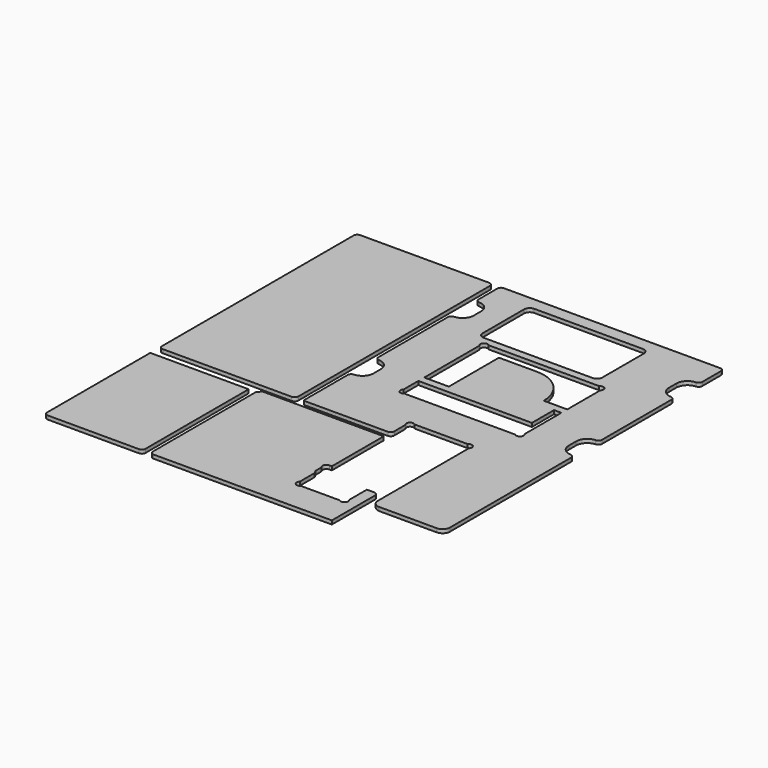
from build123d import *

# Parameters (mm, degrees)
F1_DEPTH = 1


# Not quite as in the source:
# - ends of sketch curves that miss each other by under 0.0002 mm in the source are joined


with BuildPart() as f1:
    # F0 (on Top) → F1 (new body)
    with BuildSketch(Plane.XY):
        with BuildLine():
            Line((-49.84369, 52.000023), (-49.84369, -4.632071))
            Line((-49.84369, -4.632071), (-49.84369, -12.999847))
            ThreePointArc((-49.84369, -12.999847), (-49.5508014675, -13.7069564675), (-48.843692, -13.999845))
            Line((-48.843692, -13.999845), (-13.843762, -13.999845))
            ThreePointArc((-13.843762, -13.9998449989), (-13.136642867, -13.706966133), (-12.8437640011, -12.999847))
            Line((-12.843764, -12.999847), (-12.843764, -4.632071))
            Line((-12.843764, -4.632071), (-12.843764, 52.000023))
            ThreePointArc((-12.8437640013, 52.000023), (-13.1366419884, 52.7071430116), (-13.843762, 53.0000209987))
            Line((-13.843762, 53.000021), (-48.843692, 53.000021))
            ThreePointArc((-48.843692, 53.0000209998), (-49.5508026391, 52.7071336391), (-49.8436899998, 52.000023))
        make_face()
    extrude(amount=F1_DEPTH)


with BuildPart() as f1b:
    # F0 (on Top) → F1, piece 2 (new body)
    with BuildSketch(Plane.XY):
        with BuildLine():
            Line((-48.843692, -53.000021), (-24.125936, -53.000021))
            ThreePointArc((-24.125936, -53.000021), (-23.4188315117, -52.7071274883), (-23.125938, -52.000023))
            Line((-23.125938, -52.000023), (-23.125938, -16.999839))
            Line((-23.125938, -16.999839), (-49.84369, -16.999839))
            Line((-49.84369, -16.999839), (-49.84369, -52.000023))
            ThreePointArc((-49.843689999, -52.000023), (-49.5507844797, -52.7071154797), (-48.843692, -53.000020999))
        make_face()
    extrude(amount=F1_DEPTH)


with BuildPart() as f1c:
    # F0 (on Top) → F1, piece 3 (new body)
    with BuildSketch(Plane.XY):
        with BuildLine():
            ThreePointArc((11.3220496611, -35.3140013389), (11.1054475003, -34.2240151152), (12.0297310005, -33.6070171613))
            Line((12.0297310005, -33.6070171613), (12.722098, -33.607018))
            Line((12.722098, -33.607018), (12.722098, -15.999841))
            Line((12.722098, -15.999841), (-20.125944, -15.999841))
            Line((-20.125944, -15.999841), (-21.125942, -16.999839))
            Line((-21.125942, -16.999839), (-21.125942, -52.000023))
            ThreePointArc((-21.125942, -52.000023), (-20.8330265213, -52.7071055213), (-20.125944, -53.000020997))
            Line((-20.125944, -53.000020997), (28.242006, -53.000021))
            Line((28.242006, -53.000021), (28.242006, -52.000023))
            Line((28.242006, -52.000023), (28.242006, -38.339903))
            ThreePointArc((28.242006, -38.339903), (27.9606950958, -37.6445668865), (27.2750267787, -37.3404499772))
            Line((27.2750267787, -37.3404499772), (25.221946, -37.341683))
            Line((25.221946, -37.341683), (25.221946, -43.335575))
            ThreePointArc((25.221946, -43.335575), (25.2219457726, -44.7498467726), (23.8076742274, -44.7498467726))
            Line((23.8076742274, -44.7498467726), (13.236194, -44.749847))
            ThreePointArc((13.236194, -44.749847), (11.8219222274, -44.7498467726), (11.8219222274, -43.3355752274))
            Line((11.8219222274, -43.3355752274), (11.821922, -38.348793))
            Line((11.821922, -38.348793), (11.8126693234, -38.3302876467))
            Line((11.8126693234, -38.3302876467), (11.3316786766, -37.3683063533))
            Line((11.3316786766, -37.3683063533), (11.32205, -37.349049))
            Line((11.32205, -37.349049), (11.3220496611, -35.3140013389))
        make_face()
    extrude(amount=F1_DEPTH)


with BuildPart() as f1d:
    # F0 (on Top) → F1, piece 4 (new body)
    with BuildSketch(Plane.XY):
        with BuildLine():
            Line((-9.84377, -13.814933), (12.077446, -13.814933))
            ThreePointArc((12.077446, -13.814933), (12.7580726434, -13.5084192102), (13.0368039831, -12.815951))
            Line((13.0368039831, -12.815951), (13.036804, -9.064371))
            ThreePointArc((13.036804, -9.064371), (13.0368846628, -7.6501796628), (14.4510763316, -7.6503526685))
            Line((14.4510763316, -7.6503526685), (28.82773, -7.650353))
            ThreePointArc((28.82773, -7.650353), (30.2419053372, -7.6501956628), (30.2420023393, -9.0643713393))
            Line((30.2420023393, -9.0643713393), (30.242002, -39.915465))
            ThreePointArc((30.242002, -39.915465), (30.8277878518, -41.3296751482), (32.241998, -41.915461))
            Line((32.241998, -41.915461), (47.843694, -41.915461))
            ThreePointArc((47.843694, -41.915461), (49.2579050268, -41.3296760268), (49.84369, -39.915465))
            Line((49.84369, -39.915465), (49.84369, 1.188847))
            ThreePointArc((49.84369, 1.188847), (49.5650323815, 1.8814639379), (48.8843320024, 2.1880830581))
            ThreePointArc((48.8843320024, 2.1880830581), (46.8422776076, 3.1078090407), (46.0062580004, 5.185537))
            Line((46.0062580004, 5.185537), (46.006258, 7.685405))
            ThreePointArc((46.006258, 7.685405), (46.8422117178, 9.7632741192), (48.884332003, 10.6831129264))
            ThreePointArc((48.884332003, 10.6831129264), (49.5649667808, 10.9896189332), (49.8436899878, 11.682095))
            Line((49.8436899878, 11.682095), (49.84369, 35.188779))
            ThreePointArc((49.84369, 35.188779), (49.5650387607, 35.8814020397), (48.884331999, 36.1880149755))
            ThreePointArc((48.884331999, 36.1880149755), (46.8422836938, 37.10774685), (46.0062580008, 39.185469))
            Line((46.0062580008, 39.185469), (46.006258, 41.685591))
            ThreePointArc((46.006258, 41.685591), (46.8422927104, 43.7633044161), (48.8843320031, 44.683044923))
            ThreePointArc((48.8843320031, 44.683044923), (49.5650483633, 44.9896486415), (49.8436899971, 45.682281))
            Line((49.8436899971, 45.682281), (49.84369, 52.000023))
            ThreePointArc((49.84369, 52.000023), (49.5508032248, 52.7071342248), (48.843692, 53.0000209998))
            Line((48.843692, 53.0000209998), (-9.84377, 53.000021))
            ThreePointArc((-9.84377, 53.000021), (-10.5508812248, 52.7071342248), (-10.8437679998, 52.000023))
            Line((-10.8437679998, 52.000023), (-10.843768, 45.682281))
            ThreePointArc((-10.843768, 45.682281), (-10.5651263633, 44.9896486415), (-9.8844100134, 44.6830446702))
            ThreePointArc((-9.8844100134, 44.6830446702), (-7.8423707104, 43.7633044161), (-7.0063360017, 41.685591))
            Line((-7.0063360017, 41.685591), (-7.006336, 39.185469))
            ThreePointArc((-7.006336, 39.185469), (-7.8423616938, 37.10774685), (-9.884409992, 36.1880148021))
            ThreePointArc((-9.884409992, 36.1880148021), (-10.5651167607, 35.8814020397), (-10.8437679991, 35.188779))
            Line((-10.8437679991, 35.188779), (-10.843768, 11.682095))
            ThreePointArc((-10.843768, 11.682095), (-10.5650447808, 10.9896189332), (-9.88441001, 10.683112754))
            ThreePointArc((-9.88441001, 10.683112754), (-7.8422897178, 9.7632741192), (-7.0063360028, 7.685405))
            Line((-7.0063360028, 7.685405), (-7.006336, 5.185537))
            ThreePointArc((-7.006336, 5.185537), (-7.8423556076, 3.1078090407), (-9.884409997, 2.1880829253))
            ThreePointArc((-9.884409997, 2.1880829253), (-10.5651103815, 1.8814639379), (-10.8437679998, 1.188847))
            Line((-10.8437679998, 1.188847), (-10.8437679998, -13.5675381968))
            ThreePointArc((-10.8437679998, -13.5675381968), (-10.7713077396, -13.7424727398), (-10.5963731966, -13.814933))
            Line((-10.5963731966, -13.814933), (-9.84377, -13.814933))
        make_face()
        with BuildLine():
            Line((33.38703, 8.442071), (33.38703, 15.941929))
            Line((33.38703, 15.941929), (35.387026, 15.941929))
            Line((35.387026, 15.941929), (35.387026, 3.463417))
            ThreePointArc((35.387026, 3.463417), (35.3870257726, 2.0491452274), (33.9727542274, 2.0491452274))
            Line((33.9727542274, 2.0491452274), (3.981958, 2.049145))
            ThreePointArc((3.981958, 2.049145), (2.5677996628, 2.0492586628), (2.5679396641, 3.463417336))
            Line((2.5679396641, 3.463417336), (2.56794, 8.442071))
            Line((2.56794, 8.442071), (33.38703, 8.442071))
        make_face(mode=Mode.SUBTRACT)
        with BuildLine():
            Line((35.387026, 17.941925), (29.006292, 17.941925))
            ThreePointArc((29.006292, 17.941925), (26.2238894867, 24.6594508816), (19.506438, 27.4420329985))
            Line((19.506438, 27.4420329985), (9.243822, 27.442033))
            Line((9.243822, 27.442033), (9.243822, 10.442067))
            Line((9.243822, 10.442067), (2.56794, 10.442067))
            Line((2.56794, 10.442067), (2.56794, 29.120465))
            ThreePointArc((2.56794, 29.120465), (2.5677936628, 30.5346293372), (3.9819583386, 30.5347373387))
            Line((3.9819583386, 30.5347373387), (33.972754, 30.534737))
            ThreePointArc((33.972754, 30.534737), (35.3870257726, 30.5347367726), (35.3870257726, 29.1204652274))
            Line((35.3870257726, 29.1204652274), (35.387026, 17.941925))
        make_face(mode=Mode.SUBTRACT)
        with BuildLine():
            ThreePointArc((32.0420999981, 34.064321), (31.60274582, 33.00355118), (30.541976, 32.5641970019))
            Line((30.541976, 32.564197), (1.040638, 32.564197))
            ThreePointArc((1.040638, 32.5641970082), (-0.0199740624, 33.0036345427), (-0.4592319969, 34.064321))
            Line((-0.459232, 34.064321), (-0.459232, 48.134651))
            ThreePointArc((-0.4592319965, 48.134651), (-0.0199758198, 49.1953392147), (1.040638, 49.6347749924))
            Line((1.040638, 49.634775), (30.541976, 49.634775))
            ThreePointArc((30.541976, 49.6347749978), (31.6027475774, 49.1954225774), (32.0420999978, 48.134651))
            Line((32.0421, 48.134651), (32.0421, 34.064321))
        make_face(mode=Mode.SUBTRACT)
    extrude(amount=F1_DEPTH)


solid = Compound([f1.part, f1b.part, f1c.part, f1d.part])
